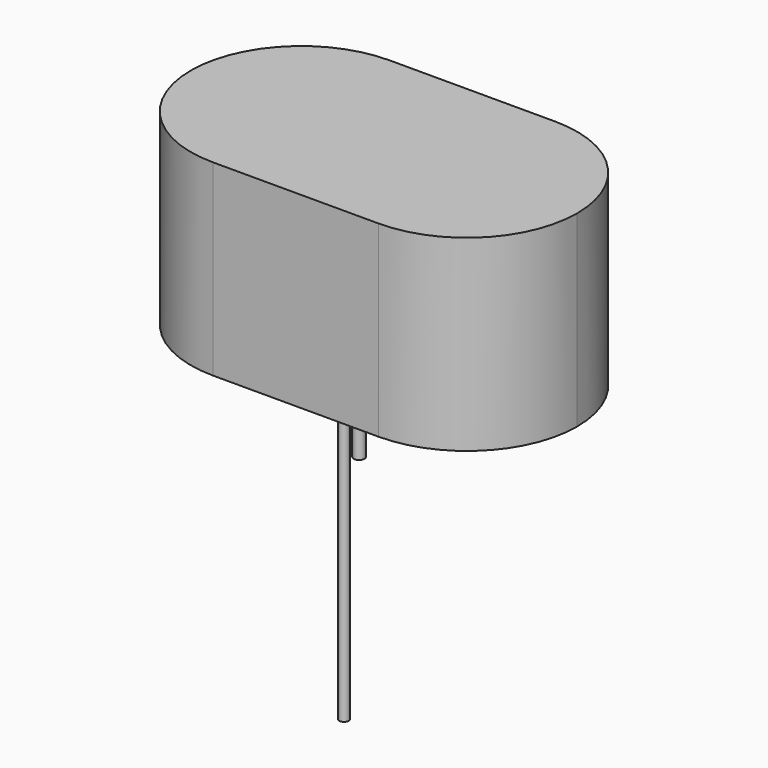
from build123d import *

# Parameters (mm, degrees)
F0_W     = 175
F0_H     = 100
F1_DEPTH = 85
F2_R     = 49.99999
F3_R     = 49.99999
F6_R     = 2.4206343252
F7_DEPTH = 15.2
F8_R     = 2.136311852
F9_DEPTH = 121.8


# Not quite as in the source:
# - a fillet or chamfer is up to 0.001 mm smaller than in the source, because OpenCascade refuses the exact size
# - the program builds the solid bodies; features that only make, move or delete a surface that nothing else refers to are left out


with BuildPart() as f1:
    # F0 (on Top) → F1 (new body)
    with BuildSketch(Plane.XY):
        with Locations((87.5, 50)):
            Rectangle(F0_W, F0_H)
    extrude(amount=F1_DEPTH)

    # F2 (radius 50 in the source; OpenCascade refuses exactly that, so slightly less here)
    f2_edges = [f1.edges().sort_by_distance(p)[0] for p in [
        (0, 0, 42.5),
        (0, 100, 42.5),
    ]]
    fillet(f2_edges, radius=F2_R)

    # F3 (radius 50 in the source; OpenCascade refuses exactly that, so slightly less here)
    f3_edges = [f1.edges().sort_by_distance(p)[0] for p in [
        (175, 100, 42.5),
        (175, 0, 42.5),
    ]]
    fillet(f3_edges, radius=F3_R)

    # F6 (on face) → F7 (join)
    with BuildSketch(Plane(origin=(0, 0, 0), x_dir=(1, 0, 0), z_dir=(0, 0, -1))):
        with Locations((111.062400043, -6.450037472)):
            Circle(F6_R)
    extrude(amount=F7_DEPTH)

    # F8 (on face) → F9 (join)
    with BuildSketch(Plane(origin=(0, 0, 0), x_dir=(1, 0, 0), z_dir=(0, 0, -1))):
        with Locations((104.4254601002, -6.2192697078)):
            Circle(F8_R)
    extrude(amount=F9_DEPTH)


solid = f1.part
